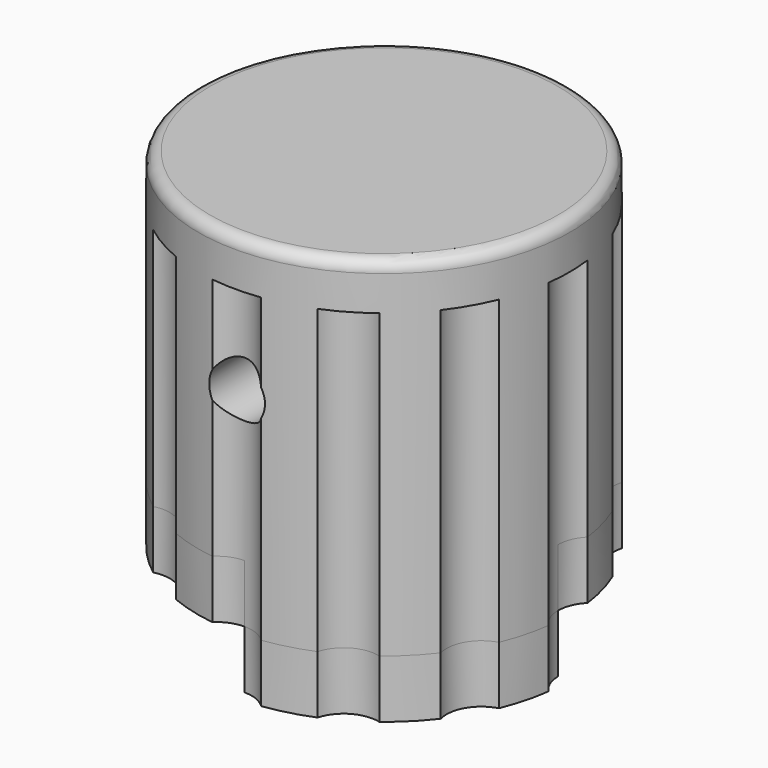
from build123d import *
from build123d import SkipClean  # not in build123d's __all__

# Parameters (mm, degrees)
F2_R      = 3.05
F3_DEPTH  = 13
F4_R      = 0.5
F5_R      = 1.2
F6_DEPTH  = 10
F7_R      = 1.5
F8_DEPTH  = 13
F10_DEPTH = 2.5
F11_DEPTH = 2.5
F13_DEPTH = 2.5


# Not quite as in the source:
# - after a boolean that leaves OpenCascade's solid faulty, fix() repairs it


with BuildPart() as f1:
    # F0 (on Front) → F1 (revolve)
    with BuildSketch(Plane.XZ):
        Polygon((-5, 0), (0, 0), (0, 15), (-8, 15), (-8, 0), align=None)
    revolve(axis=Axis((0, 0, -3.6677676575), (0, 0, -1)))

    # F2 (on face) → F3 (cut)
    with BuildSketch(Plane(origin=(0, 0, 0), x_dir=(1, 0, 0), z_dir=(0, 0, -1))):
        Circle(F2_R)
    extrude(amount=-F3_DEPTH, mode=Mode.SUBTRACT)

    # F4
    f4_edges = [f1.edges().sort_by_distance(p)[0] for p in [
        (8, 0, 15),
    ]]
    fillet(f4_edges, radius=F4_R)

    # F5 (on Front) → F6 (cut)
    with BuildSketch(Plane.XZ):
        with Locations((0, 9)):
            Circle(F5_R)
    extrude(amount=F6_DEPTH, mode=Mode.SUBTRACT)

    # F7 (on face) → F8 (cut)
    with BuildSketch(Plane(origin=(0, 0, 0), x_dir=(1, 0, 0), z_dir=(0, 0, -1))):
        with Locations((-9, 0)):
            Circle(F7_R)
        with Locations((-7.7942286341, -4.5)):
            Circle(F7_R)
        with Locations((-4.5, -7.7942286341)):
            Circle(F7_R)
        with Locations((0, -9)):
            Circle(F7_R)
        with Locations((4.5, -7.7942286341)):
            Circle(F7_R)
        with Locations((7.7942286341, -4.5)):
            Circle(F7_R)
        with Locations((9, 0)):
            Circle(F7_R)
        with Locations((7.7942286341, 4.5)):
            Circle(F7_R)
        with Locations((4.5, 7.7942286341)):
            Circle(F7_R)
        with Locations((0, 9)):
            Circle(F7_R)
        with Locations((-4.5, 7.7942286341)):
            Circle(F7_R)
        with Locations((-7.7942286341, 4.5)):
            Circle(F7_R)
    extrude(amount=-F8_DEPTH, mode=Mode.SUBTRACT)

    # F9 (on face) → F10 (cut)
    with BuildSketch(Plane(origin=(0, 0, 0), x_dir=(1, 0, 0), z_dir=(0, 0, -1))):
        with BuildLine():
            Line((8, 0), (0, 0))
            Line((0, 0), (0, 8))
            ThreePointArc((0, 8), (-5.6568542495, -5.6568542495), (8, 0))
        make_face()
    extrude(amount=-F10_DEPTH, mode=Mode.SUBTRACT)

    # F10_face (on face) + F1_face (on face) → F11 (join)
    with BuildSketch(Plane(origin=(-1.2304392028, 1.2304392022, 2.5), x_dir=(1, 0, 0), z_dir=(0, 0, -1))):
        with BuildLine():
            Line((8.7304392028, 1.2304392022), (4.2804392028, 1.2304392022))
            ThreePointArc((4.2804392028, 1.2304392022), (-0.9262364799, -0.9262364804), (1.2304392028, 4.2804392022))
            Line((1.2304392028, 4.2804392022), (1.2304392028, 8.7304392022))
            ThreePointArc((1.2304392028, 8.7304392022), (0.6621816316, 8.8422449317), (0.1786366634, 9.1609947585))
            ThreePointArc((0.1786366641, 9.1609947578), (-0.8401131581, 8.9578458126), (-1.8239508568, 8.6244030488))
            ThreePointArc((-1.8239508568, 8.6244030488), (-2.5195607972, 7.7256297306), (-3.6457262932, 7.5726005102))
            ThreePointArc((-3.6457262932, 7.5726005102), (-4.4264150467, 6.8872934517), (-5.1117221052, 6.1066046982))
            ThreePointArc((-5.1117221052, 6.1066046982), (-5.2647513256, 4.9804392022), (-6.1635246438, 4.2848292618))
            ThreePointArc((-6.1635246438, 4.2848292618), (-6.4969674076, 3.3009915631), (-6.7001163528, 2.2822417409))
            ThreePointArc((-6.7001163528, 2.2822417409), (-6.2695607972, 1.2304392022), (-6.7001163528, 0.1786366636))
            ThreePointArc((-6.7001163528, 0.1786366636), (-6.4969674076, -0.8401131586), (-6.1635246438, -1.8239508573))
            ThreePointArc((-6.1635246438, -1.8239508573), (-5.2647513256, -2.5195607978), (-5.1117221052, -3.6457262937))
            ThreePointArc((-5.1117221052, -3.6457262937), (-4.4264150467, -4.4264150472), (-3.6457262932, -5.1117221057))
            ThreePointArc((-3.6457262932, -5.1117221057), (-2.5195607972, -5.2647513261), (-1.8239508568, -6.1635246443))
            ThreePointArc((-1.8239508568, -6.1635246443), (-0.8401131581, -6.4969674081), (0.1786366641, -6.7001163533))
            ThreePointArc((0.1786366641, -6.7001163533), (1.2304392028, -6.2695607978), (2.2822417414, -6.7001163533))
            ThreePointArc((2.2822417414, -6.7001163533), (3.3009915636, -6.4969674081), (4.2848292623, -6.1635246443))
            ThreePointArc((4.2848292623, -6.1635246443), (4.9804392028, -5.2647513261), (6.1066046987, -5.1117221057))
            ThreePointArc((6.1066046987, -5.1117221057), (6.8872934522, -4.4264150472), (7.5726005107, -3.6457262937))
            ThreePointArc((7.5726005107, -3.6457262937), (7.7256297311, -2.5195607978), (8.6244030493, -1.8239508573))
            ThreePointArc((8.6244030493, -1.8239508573), (8.9578458131, -0.8401131586), (9.1609947583, 0.1786366636))
            ThreePointArc((9.1609947583, 0.1786366636), (8.842244932, 0.6621816315), (8.7304392028, 1.2304392022))
        make_face()
    with BuildSketch(Plane(origin=(0, 0, 0), x_dir=(1, 0, 0), z_dir=(0, 0, -1))):
        with BuildLine():
            ThreePointArc((1.0518025386, 7.9305555556), (0.5682575707, 7.6118057293), (0, 7.5))
            Line((0, 7.5), (0, 3.05))
            ThreePointArc((0, 3.05), (2.1566756826, 2.1566756826), (3.05, 0))
            Line((3.05, 0), (7.5, 0))
            ThreePointArc((7.5, 0), (7.6118057293, 0.5682575707), (7.9305555556, 1.0518025386))
            ThreePointArc((7.9305555556, 1.0518025386), (7.7274066103, 2.0705523608), (7.3939638465, 3.0543900596))
            ThreePointArc((7.3939638465, 3.0543900596), (6.4951905284, 3.75), (6.3421613079, 4.876165496))
            ThreePointArc((6.3421613079, 4.876165496), (5.6568542495, 5.6568542495), (4.876165496, 6.3421613079))
            ThreePointArc((4.876165496, 6.3421613079), (3.75, 6.4951905284), (3.0543900596, 7.3939638465))
            ThreePointArc((3.0543900596, 7.3939638465), (2.0705523608, 7.7274066103), (1.0518025386, 7.9305555556))
        make_face()
    with SkipClean():  # cleaning this boolean's faces spoils the solid; the shape is the same uncleaned
        extrude(amount=F11_DEPTH)

    # F12 (on face) → F13 (cut)
    with BuildSketch(Plane(origin=(0, 0, -2.5), x_dir=(1, 0, 0), z_dir=(0, 0, -1))):
        with BuildLine():
            ThreePointArc((0, 3.05), (2.1566756826, 2.1566756826), (3.05, 0))
            Line((3.05, 0), (5.35, 0))
            ThreePointArc((5.35, 0), (3.7410791492, 3.7410791492), (0, 5.35))
            Line((0, 5.35), (0, 3.05))
        make_face()
    extrude(amount=-F13_DEPTH, mode=Mode.SUBTRACT)

    add(f1.part.fix(), mode=Mode.REPLACE)


solid = f1.part
